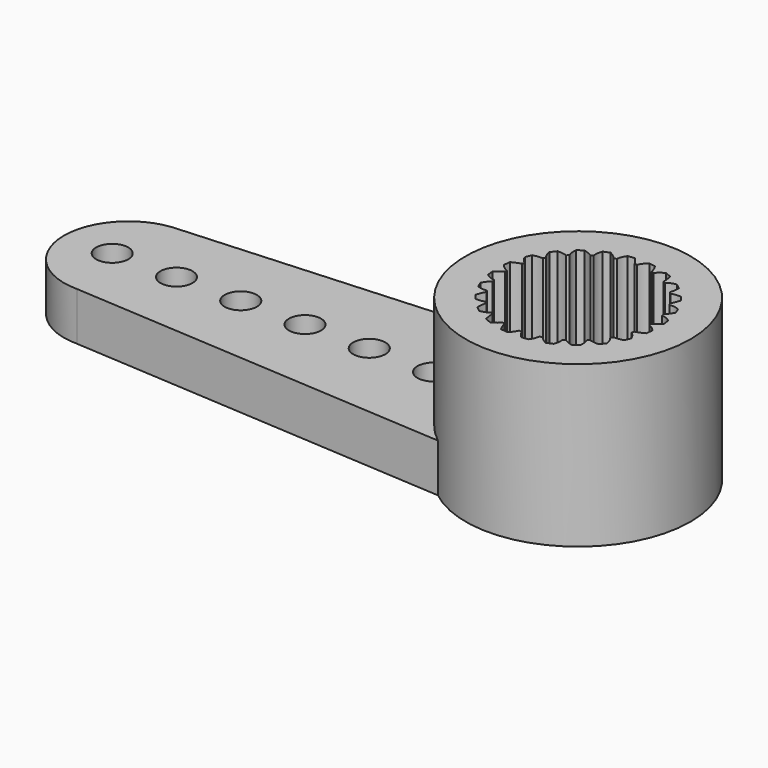
from build123d import *

# Parameters (mm, degrees)
F0_R     = 0.5
F0_R_2   = 1
F1_DEPTH = 1.5
F2_DEPTH = 5
F3_R     = 2.375
F4_DEPTH = 1
F6_DEPTH = 2.75


# Not quite as in the source:
# - a feature names something its author has since deleted; it is built from what else it names


with BuildPart() as f1:
    # F0 (on Top) → F1 (new body)
    with BuildSketch(Plane.XY):
        with BuildLine():
            ThreePointArc((-2.1650635095, -2.75), (-3.5, 0), (-2.1650635095, 2.75))
            Line((-2.1650635095, 2.75), (-14, 2))
            ThreePointArc((-14, 2), (-12.5857864376, 1.4142135624), (-12, 0))
            ThreePointArc((-12, 0), (-12.5857864376, -1.4142135624), (-14, -2))
            Line((-14, -2), (-2.1650635095, -2.75))
        make_face()
        with Locations((-10.5, 0)):
            Circle(F0_R, mode=Mode.SUBTRACT)
        with Locations((-8.5, 0)):
            Circle(F0_R, mode=Mode.SUBTRACT)
        with Locations((-6.5, 0)):
            Circle(F0_R, mode=Mode.SUBTRACT)
        with Locations((-4.5, 0)):
            Circle(F0_R, mode=Mode.SUBTRACT)
        with BuildLine():
            ThreePointArc((-2.1650635095, -2.75), (1.5284432794, -3.148628454), (3.5, 0))
            ThreePointArc((3.5, 0), (1.5284432794, 3.148628454), (-2.1650635095, 2.75))
            ThreePointArc((-2.1650635095, 2.75), (-3.5, 0), (-2.1650635095, -2.75))
        make_face()
        Circle(F0_R_2, mode=Mode.SUBTRACT)
        with BuildLine():
            ThreePointArc((-12, 0), (-12.5857864376, 1.4142135624), (-14, 2))
            ThreePointArc((-14, 2), (-16, 0), (-14, -2))
            ThreePointArc((-14, -2), (-12.5857864376, -1.4142135624), (-12, 0))
        make_face()
        with Locations((-14.5, 0)):
            Circle(F0_R, mode=Mode.SUBTRACT)
        with Locations((-12.5, 0)):
            Circle(F0_R, mode=Mode.SUBTRACT)
    extrude(amount=F1_DEPTH)

    # F0 (on Top) → F2 (join)
    with BuildSketch(Plane.XY):
        with BuildLine():
            ThreePointArc((-2.1650635095, -2.75), (1.5284432794, -3.148628454), (3.5, 0))
            ThreePointArc((3.5, 0), (1.5284432794, 3.148628454), (-2.1650635095, 2.75))
            ThreePointArc((-2.1650635095, 2.75), (-3.5, 0), (-2.1650635095, -2.75))
        make_face()
        Circle(F0_R_2, mode=Mode.SUBTRACT)
    extrude(amount=F2_DEPTH)

    # F3 (on face) → F4 (cut)
    with BuildSketch(Plane.XY):
        Circle(F3_R)
    extrude(amount=F4_DEPTH, mode=Mode.SUBTRACT)

    # F5 (on face) → F6 (cut)
    with BuildSketch(Plane.XY.offset(5)):
        with BuildLine():
            ThreePointArc((2.2496444163, -0.04), (2.2499111023, -0.0200007902), (2.25, 0))
            ThreePointArc((2.25, 0), (2.2499111023, 0.0200007902), (2.2496444163, 0.04))
            ThreePointArc((2.2496444163, 0.04), (2.2307509381, 0.2936839325), (2.1833424035, 0.5436137866))
            ThreePointArc((2.1833424035, 0.5436137866), (2.1733331092, 0.5823428515), (2.1626368799, 0.6208878527))
            ThreePointArc((2.1626368799, 0.6208878527), (2.0787289482, 0.8610377228), (1.968249214, 1.090181192))
            ThreePointArc((1.968249214, 1.090181192), (1.9485571585, 1.125), (1.928249214, 1.1594632243))
            ThreePointArc((1.928249214, 1.1594632243), (1.7850450157, 1.3697132153), (1.6190230933, 1.5624545508))
            ThreePointArc((1.6190230933, 1.5624545508), (1.5909902577, 1.5909902577), (1.5624545508, 1.6190230933))
            ThreePointArc((1.5624545508, 1.6190230933), (1.3697132153, 1.7850450157), (1.1594632243, 1.928249214))
            ThreePointArc((1.1594632243, 1.928249214), (1.125, 1.9485571585), (1.090181192, 1.968249214))
            ThreePointArc((1.090181192, 1.968249214), (0.8610377228, 2.0787289482), (0.6208878527, 2.1626368799))
            ThreePointArc((0.6208878527, 2.1626368799), (0.5823428515, 2.1733331092), (0.5436137866, 2.1833424035))
            ThreePointArc((0.5436137866, 2.1833424035), (0.2936839325, 2.2307509381), (0.04, 2.2496444163))
            ThreePointArc((0.04, 2.2496444163), (0, 2.25), (-0.04, 2.2496444163))
            ThreePointArc((-0.04, 2.2496444163), (-0.2936839325, 2.2307509381), (-0.5436137866, 2.1833424035))
            ThreePointArc((-0.5436137866, 2.1833424035), (-0.5823428515, 2.1733331092), (-0.6208878527, 2.1626368799))
            ThreePointArc((-0.6208878527, 2.1626368799), (-0.8610377228, 2.0787289482), (-1.090181192, 1.968249214))
            ThreePointArc((-1.090181192, 1.968249214), (-1.125, 1.9485571585), (-1.1594632243, 1.928249214))
            ThreePointArc((-1.1594632243, 1.928249214), (-1.3697132153, 1.7850450157), (-1.5624545508, 1.6190230933))
            ThreePointArc((-1.5624545508, 1.6190230933), (-1.5909902577, 1.5909902577), (-1.6190230933, 1.5624545508))
            ThreePointArc((-1.6190230933, 1.5624545508), (-1.7850450157, 1.3697132153), (-1.928249214, 1.1594632243))
            ThreePointArc((-1.928249214, 1.1594632243), (-1.9485571585, 1.125), (-1.968249214, 1.090181192))
            ThreePointArc((-1.968249214, 1.090181192), (-2.0787289482, 0.8610377228), (-2.1626368799, 0.6208878527))
            ThreePointArc((-2.1626368799, 0.6208878527), (-2.1733331092, 0.5823428515), (-2.1833424035, 0.5436137866))
            ThreePointArc((-2.1833424035, 0.5436137866), (-2.2307509381, 0.2936839325), (-2.2496444163, 0.04))
            ThreePointArc((-2.2496444163, 0.04), (-2.25, 0), (-2.2496444163, -0.04))
            ThreePointArc((-2.2496444163, -0.04), (-2.2307509381, -0.2936839325), (-2.1833424035, -0.5436137866))
            ThreePointArc((-2.1833424035, -0.5436137866), (-2.1733331092, -0.5823428515), (-2.1626368799, -0.6208878527))
            ThreePointArc((-2.1626368799, -0.6208878527), (-2.0787289482, -0.8610377228), (-1.968249214, -1.090181192))
            ThreePointArc((-1.968249214, -1.090181192), (-1.9485571585, -1.125), (-1.928249214, -1.1594632243))
            ThreePointArc((-1.928249214, -1.1594632243), (-1.7850450157, -1.3697132153), (-1.6190230933, -1.5624545508))
            ThreePointArc((-1.6190230933, -1.5624545508), (-1.5909902577, -1.5909902577), (-1.5624545508, -1.6190230933))
            ThreePointArc((-1.5624545508, -1.6190230933), (-1.3697132153, -1.7850450157), (-1.1594632243, -1.928249214))
            ThreePointArc((-1.1594632243, -1.928249214), (-1.125, -1.9485571585), (-1.090181192, -1.968249214))
            ThreePointArc((-1.090181192, -1.968249214), (-0.8610377228, -2.0787289482), (-0.6208878527, -2.1626368799))
            ThreePointArc((-0.6208878527, -2.1626368799), (-0.5823428515, -2.1733331092), (-0.5436137866, -2.1833424035))
            ThreePointArc((-0.5436137866, -2.1833424035), (-0.2936839325, -2.2307509381), (-0.04, -2.2496444163))
            ThreePointArc((-0.04, -2.2496444163), (0, -2.25), (0.04, -2.2496444163))
            ThreePointArc((0.04, -2.2496444163), (0.2936839325, -2.2307509381), (0.5436137866, -2.1833424035))
            ThreePointArc((0.5436137866, -2.1833424035), (0.5823428515, -2.1733331092), (0.6208878527, -2.1626368799))
            ThreePointArc((0.6208878527, -2.1626368799), (0.8610377228, -2.0787289482), (1.090181192, -1.968249214))
            ThreePointArc((1.090181192, -1.968249214), (1.125, -1.9485571585), (1.1594632243, -1.928249214))
            ThreePointArc((1.1594632243, -1.928249214), (1.3697132153, -1.7850450157), (1.5624545508, -1.6190230933))
            ThreePointArc((1.5624545508, -1.6190230933), (1.5909902577, -1.5909902577), (1.6190230933, -1.5624545508))
            ThreePointArc((1.6190230933, -1.5624545508), (1.7850450157, -1.3697132153), (1.928249214, -1.1594632243))
            ThreePointArc((1.928249214, -1.1594632243), (1.9485571585, -1.125), (1.968249214, -1.090181192))
            ThreePointArc((1.968249214, -1.090181192), (2.0787289482, -0.8610377228), (2.1626368799, -0.6208878527))
            ThreePointArc((2.1626368799, -0.6208878527), (2.1733331092, -0.5823428515), (2.1833424035, -0.5436137866))
            ThreePointArc((2.1833424035, -0.5436137866), (2.2307509381, -0.2936839325), (2.2496444163, -0.04))
        make_face()
        with BuildLine():
            ThreePointArc((2.1833424035, 0.5436137866), (2.2307509381, 0.2936839325), (2.2496444163, 0.04))
            ThreePointArc((2.2496444163, 0.04), (2.376347735, 0.1239325273), (2.4898544134, 0.225))
            ThreePointArc((2.4898544134, 0.225), (2.47674458, 0.3260696098), (2.4632489668, 0.4270884308))
            ThreePointArc((2.4632489668, 0.4270884308), (2.3313772515, 0.5047639091), (2.1833424035, 0.5436137866))
        make_face()
        with BuildLine():
            ThreePointArc((2.4898544134, -0.225), (2.382580011, -0.115840338), (2.2496444163, -0.04))
            ThreePointArc((2.2496444163, -0.04), (2.2307509381, -0.2936839325), (2.1833424035, -0.5436137866))
            ThreePointArc((2.1833424035, -0.5436137866), (2.3274517478, -0.4953344228), (2.4632489668, -0.4270884308))
            ThreePointArc((2.4632489668, -0.4270884308), (2.47674458, -0.3260696098), (2.4898544134, -0.225))
        make_face()
        with BuildLine():
            ThreePointArc((1.968249214, 1.090181192), (2.0787289482, 0.8610377228), (2.1626368799, 0.6208878527))
            ThreePointArc((2.1626368799, 0.6208878527), (2.2632995511, 0.7347536804), (2.3467803965, 0.8617550526))
            ThreePointArc((2.3467803965, 0.8617550526), (2.3079585298, 0.9559877245), (2.2687771737, 1.0500714909))
            ThreePointArc((2.2687771737, 1.0500714909), (2.1212949851, 1.09096933), (1.968249214, 1.090181192))
        make_face()
        with BuildLine():
            ThreePointArc((2.3467803965, -0.8617550526), (2.2714138802, -0.7285502576), (2.1626368799, -0.6208878527))
            ThreePointArc((2.1626368799, -0.6208878527), (2.0787289482, -0.8610377228), (1.968249214, -1.090181192))
            ThreePointArc((1.968249214, -1.090181192), (2.1199437704, -1.0808451505), (2.2687771737, -1.0500714909))
            ThreePointArc((2.2687771737, -1.0500714909), (2.3079585298, -0.9559877245), (2.3467803965, -0.8617550526))
        make_face()
        with BuildLine():
            ThreePointArc((1.6190230933, 1.5624545508), (1.7850450157, 1.3697132153), (1.928249214, 1.1594632243))
            ThreePointArc((1.928249214, 1.1594632243), (1.9960112431, 1.2955025845), (2.0437771737, 1.4397829226))
            ThreePointArc((2.0437771737, 1.4397829226), (1.98188892, 1.5207568555), (1.9196919657, 1.6014939141))
            ThreePointArc((1.9196919657, 1.6014939141), (1.7666499711, 1.602826994), (1.6190230933, 1.5624545508))
        make_face()
        with BuildLine():
            ThreePointArc((2.0437771737, -1.4397829226), (2.0054546471, -1.291610681), (1.928249214, -1.1594632243))
            ThreePointArc((1.928249214, -1.1594632243), (1.7850450157, -1.3697132153), (1.6190230933, -1.5624545508))
            ThreePointArc((1.6190230933, -1.5624545508), (1.7679651283, -1.5926980674), (1.9196919657, -1.6014939141))
            ThreePointArc((1.9196919657, -1.6014939141), (1.98188892, -1.5207568555), (2.0437771737, -1.4397829226))
        make_face()
        with BuildLine():
            ThreePointArc((1.1594632243, 1.928249214), (1.3697132153, 1.7850450157), (1.5624545508, 1.6190230933))
            ThreePointArc((1.5624545508, 1.6190230933), (1.5926980674, 1.7679651283), (1.6014939141, 1.9196919657))
            ThreePointArc((1.6014939141, 1.9196919657), (1.5207568555, 1.98188892), (1.4397829226, 2.0437771737))
            ThreePointArc((1.4397829226, 2.0437771737), (1.291610681, 2.0054546471), (1.1594632243, 1.928249214))
        make_face()
        with BuildLine():
            ThreePointArc((1.6014939141, -1.9196919657), (1.602826994, -1.7666499711), (1.5624545508, -1.6190230933))
            ThreePointArc((1.5624545508, -1.6190230933), (1.3697132153, -1.7850450157), (1.1594632243, -1.928249214))
            ThreePointArc((1.1594632243, -1.928249214), (1.2955025845, -1.9960112431), (1.4397829226, -2.0437771737))
            ThreePointArc((1.4397829226, -2.0437771737), (1.5207568555, -1.98188892), (1.6014939141, -1.9196919657))
        make_face()
        with BuildLine():
            ThreePointArc((0.6208878527, 2.1626368799), (0.8610377228, 2.0787289482), (1.090181192, 1.968249214))
            ThreePointArc((1.090181192, 1.968249214), (1.0808451505, 2.1199437704), (1.0500714909, 2.2687771737))
            ThreePointArc((1.0500714909, 2.2687771737), (0.9559877245, 2.3079585298), (0.8617550526, 2.3467803965))
            ThreePointArc((0.8617550526, 2.3467803965), (0.7285502576, 2.2714138802), (0.6208878527, 2.1626368799))
        make_face()
        with BuildLine():
            ThreePointArc((1.0500714909, -2.2687771737), (1.09096933, -2.1212949851), (1.090181192, -1.968249214))
            ThreePointArc((1.090181192, -1.968249214), (0.8610377228, -2.0787289482), (0.6208878527, -2.1626368799))
            ThreePointArc((0.6208878527, -2.1626368799), (0.7347536804, -2.2632995511), (0.8617550526, -2.3467803965))
            ThreePointArc((0.8617550526, -2.3467803965), (0.9559877245, -2.3079585298), (1.0500714909, -2.2687771737))
        make_face()
        with BuildLine():
            ThreePointArc((0.04, 2.2496444163), (0.2936839325, 2.2307509381), (0.5436137866, 2.1833424035))
            ThreePointArc((0.5436137866, 2.1833424035), (0.4953344228, 2.3274517478), (0.4270884308, 2.4632489668))
            ThreePointArc((0.4270884308, 2.4632489668), (0.3260696098, 2.47674458), (0.225, 2.4898544134))
            ThreePointArc((0.225, 2.4898544134), (0.115840338, 2.382580011), (0.04, 2.2496444163))
        make_face()
        with BuildLine():
            ThreePointArc((0.4270884308, -2.4632489668), (0.5047639091, -2.3313772515), (0.5436137866, -2.1833424035))
            ThreePointArc((0.5436137866, -2.1833424035), (0.2936839325, -2.2307509381), (0.04, -2.2496444163))
            ThreePointArc((0.04, -2.2496444163), (0.1239325273, -2.376347735), (0.225, -2.4898544134))
            ThreePointArc((0.225, -2.4898544134), (0.3260696098, -2.47674458), (0.4270884308, -2.4632489668))
        make_face()
        with BuildLine():
            ThreePointArc((-0.5436137866, 2.1833424035), (-0.2936839325, 2.2307509381), (-0.04, 2.2496444163))
            ThreePointArc((-0.04, 2.2496444163), (-0.1239325273, 2.376347735), (-0.225, 2.4898544134))
            ThreePointArc((-0.225, 2.4898544134), (-0.3260696098, 2.47674458), (-0.4270884308, 2.4632489668))
            ThreePointArc((-0.4270884308, 2.4632489668), (-0.5047639091, 2.3313772515), (-0.5436137866, 2.1833424035))
        make_face()
        with BuildLine():
            ThreePointArc((-0.225, -2.4898544134), (-0.115840338, -2.382580011), (-0.04, -2.2496444163))
            ThreePointArc((-0.04, -2.2496444163), (-0.2936839325, -2.2307509381), (-0.5436137866, -2.1833424035))
            ThreePointArc((-0.5436137866, -2.1833424035), (-0.4953344228, -2.3274517478), (-0.4270884308, -2.4632489668))
            ThreePointArc((-0.4270884308, -2.4632489668), (-0.3260696098, -2.47674458), (-0.225, -2.4898544134))
        make_face()
        with BuildLine():
            ThreePointArc((-1.090181192, 1.968249214), (-0.8610377228, 2.0787289482), (-0.6208878527, 2.1626368799))
            ThreePointArc((-0.6208878527, 2.1626368799), (-0.7347536804, 2.2632995511), (-0.8617550526, 2.3467803965))
            ThreePointArc((-0.8617550526, 2.3467803965), (-0.9559877245, 2.3079585298), (-1.0500714909, 2.2687771737))
            ThreePointArc((-1.0500714909, 2.2687771737), (-1.09096933, 2.1212949851), (-1.090181192, 1.968249214))
        make_face()
        with BuildLine():
            ThreePointArc((-0.8617550526, -2.3467803965), (-0.7285502576, -2.2714138802), (-0.6208878527, -2.1626368799))
            ThreePointArc((-0.6208878527, -2.1626368799), (-0.8610377228, -2.0787289482), (-1.090181192, -1.968249214))
            ThreePointArc((-1.090181192, -1.968249214), (-1.0808451505, -2.1199437704), (-1.0500714909, -2.2687771737))
            ThreePointArc((-1.0500714909, -2.2687771737), (-0.9559877245, -2.3079585298), (-0.8617550526, -2.3467803965))
        make_face()
        with BuildLine():
            ThreePointArc((-1.5624545508, 1.6190230933), (-1.3697132153, 1.7850450157), (-1.1594632243, 1.928249214))
            ThreePointArc((-1.1594632243, 1.928249214), (-1.2955025845, 1.9960112431), (-1.4397829226, 2.0437771737))
            ThreePointArc((-1.4397829226, 2.0437771737), (-1.5207568555, 1.98188892), (-1.6014939141, 1.9196919657))
            ThreePointArc((-1.6014939141, 1.9196919657), (-1.602826994, 1.7666499711), (-1.5624545508, 1.6190230933))
        make_face()
        with BuildLine():
            ThreePointArc((-1.4397829226, -2.0437771737), (-1.291610681, -2.0054546471), (-1.1594632243, -1.928249214))
            ThreePointArc((-1.1594632243, -1.928249214), (-1.3697132153, -1.7850450157), (-1.5624545508, -1.6190230933))
            ThreePointArc((-1.5624545508, -1.6190230933), (-1.5926980674, -1.7679651283), (-1.6014939141, -1.9196919657))
            ThreePointArc((-1.6014939141, -1.9196919657), (-1.5207568555, -1.98188892), (-1.4397829226, -2.0437771737))
        make_face()
        with BuildLine():
            ThreePointArc((-1.928249214, 1.1594632243), (-1.7850450157, 1.3697132153), (-1.6190230933, 1.5624545508))
            ThreePointArc((-1.6190230933, 1.5624545508), (-1.7679651283, 1.5926980674), (-1.9196919657, 1.6014939141))
            ThreePointArc((-1.9196919657, 1.6014939141), (-1.98188892, 1.5207568555), (-2.0437771737, 1.4397829226))
            ThreePointArc((-2.0437771737, 1.4397829226), (-2.0054546471, 1.291610681), (-1.928249214, 1.1594632243))
        make_face()
        with BuildLine():
            ThreePointArc((-1.9196919657, -1.6014939141), (-1.7666499711, -1.602826994), (-1.6190230933, -1.5624545508))
            ThreePointArc((-1.6190230933, -1.5624545508), (-1.7850450157, -1.3697132153), (-1.928249214, -1.1594632243))
            ThreePointArc((-1.928249214, -1.1594632243), (-1.9960112431, -1.2955025845), (-2.0437771737, -1.4397829226))
            ThreePointArc((-2.0437771737, -1.4397829226), (-1.98188892, -1.5207568555), (-1.9196919657, -1.6014939141))
        make_face()
        with BuildLine():
            ThreePointArc((-2.1626368799, 0.6208878527), (-2.0787289482, 0.8610377228), (-1.968249214, 1.090181192))
            ThreePointArc((-1.968249214, 1.090181192), (-2.1199437704, 1.0808451505), (-2.2687771737, 1.0500714909))
            ThreePointArc((-2.2687771737, 1.0500714909), (-2.3079585298, 0.9559877245), (-2.3467803965, 0.8617550526))
            ThreePointArc((-2.3467803965, 0.8617550526), (-2.2714138802, 0.7285502576), (-2.1626368799, 0.6208878527))
        make_face()
        with BuildLine():
            ThreePointArc((-2.2687771737, -1.0500714909), (-2.1212949851, -1.09096933), (-1.968249214, -1.090181192))
            ThreePointArc((-1.968249214, -1.090181192), (-2.0787289482, -0.8610377228), (-2.1626368799, -0.6208878527))
            ThreePointArc((-2.1626368799, -0.6208878527), (-2.2632995511, -0.7347536804), (-2.3467803965, -0.8617550526))
            ThreePointArc((-2.3467803965, -0.8617550526), (-2.3079585298, -0.9559877245), (-2.2687771737, -1.0500714909))
        make_face()
        with BuildLine():
            ThreePointArc((-2.2496444163, 0.04), (-2.2307509381, 0.2936839325), (-2.1833424035, 0.5436137866))
            ThreePointArc((-2.1833424035, 0.5436137866), (-2.3274517478, 0.4953344228), (-2.4632489668, 0.4270884308))
            ThreePointArc((-2.4632489668, 0.4270884308), (-2.47674458, 0.3260696098), (-2.4898544134, 0.225))
            ThreePointArc((-2.4898544134, 0.225), (-2.382580011, 0.115840338), (-2.2496444163, 0.04))
        make_face()
        with BuildLine():
            ThreePointArc((-2.4632489668, -0.4270884308), (-2.3313772515, -0.5047639091), (-2.1833424035, -0.5436137866))
            ThreePointArc((-2.1833424035, -0.5436137866), (-2.2307509381, -0.2936839325), (-2.2496444163, -0.04))
            ThreePointArc((-2.2496444163, -0.04), (-2.376347735, -0.1239325273), (-2.4898544134, -0.225))
            ThreePointArc((-2.4898544134, -0.225), (-2.47674458, -0.3260696098), (-2.4632489668, -0.4270884308))
        make_face()
    extrude(amount=-F6_DEPTH, mode=Mode.SUBTRACT)


solid = f1.part
